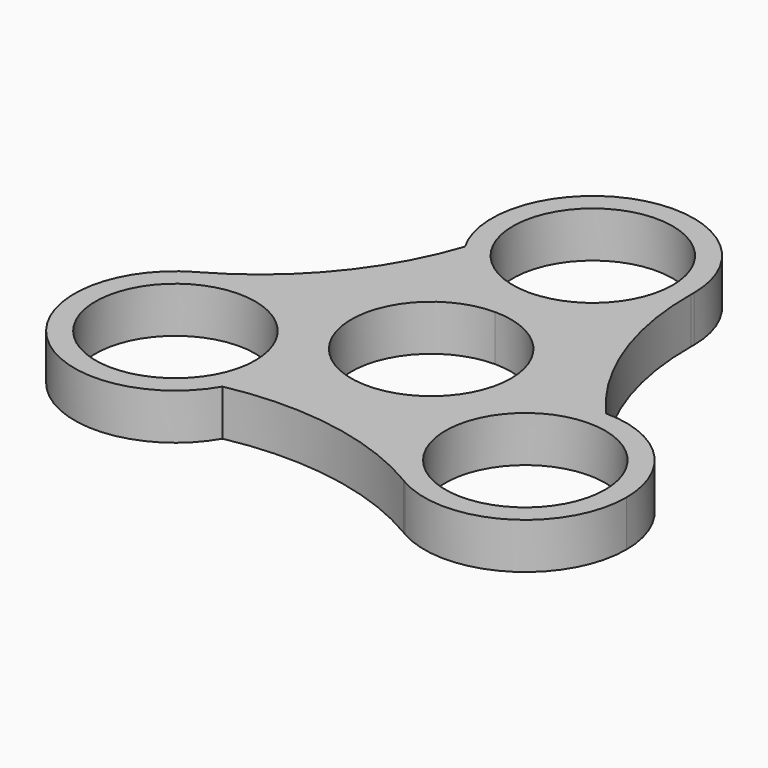
from build123d import *

# Parameters (mm, degrees)
F1_R     = 11.049
F2_DEPTH = 6.35


with BuildPart() as f2:
    # F1 (on face) → F2 (new body)
    with BuildSketch(Plane.XY):
        with BuildLine():
            ThreePointArc((13.9621660883, 27.472220007), (13.9654123098, 27.7061212363), (13.97, 27.94))
            ThreePointArc((13.97, 27.94), (-3.6157020601, 41.4339837933), (-12.0983748909, 20.955))
            ThreePointArc((-12.0983748909, 20.955), (-6.9849999951, 15.8416251063), (1.14e-08, 13.97))
            ThreePointArc((1.14e-08, 13.97), (9.7114883941, 17.8976948278), (13.9621660883, 27.472220007))
        make_face()
        with BuildLine():
            ThreePointArc((11.049, 27.94), (7.8128228253, 20.1271771747), (0, 16.891))
            ThreePointArc((0, 16.891), (-7.8128228253, 35.7528228253), (11.049, 27.94))
        make_face(mode=Mode.SUBTRACT)
        with BuildLine():
            ThreePointArc((1.14e-08, 13.97), (-6.9849999951, 15.8416251063), (-12.0983748909, 20.955))
            ThreePointArc((-12.0983748909, 20.955), (-19.3348001595, 7.9193573575), (-30.7727234686, -1.6445194791))
            ThreePointArc((-30.7727234686, -1.6445194791), (-20.3556031034, -0.5384516084), (-12.0983754336, -6.98499906))
            ThreePointArc((-12.0983754336, -6.98499906), (-12.0983746167, 6.9850004749), (1.14e-08, 13.97))
        make_face()
        with BuildLine():
            ThreePointArc((24.1967497817, 0), (16.525764733, 12.7847494365), (13.9621660883, 27.472220007))
            ThreePointArc((13.9621660883, 27.472220007), (9.7114883941, 17.8976948278), (1.14e-08, 13.97))
            ThreePointArc((1.14e-08, 13.97), (9.8782817372, 9.8782817292), (13.97, 0))
            ThreePointArc((13.97, 0), (13.4939839355, -3.6157015292), (12.0983754405, -6.984999048))
            ThreePointArc((12.0983754405, -6.984999048), (17.2117502577, -1.8716248343), (24.1967497817, 0))
        make_face()
        with BuildLine():
            ThreePointArc((13.97, 0), (9.8782817372, 9.8782817292), (1.14e-08, 13.97))
            ThreePointArc((1.14e-08, 13.97), (-12.0983746167, 6.9850004749), (-12.0983754336, -6.98499906))
            ThreePointArc((-12.0983754336, -6.98499906), (6.9e-09, -13.97), (12.0983754405, -6.984999048))
            ThreePointArc((12.0983754405, -6.984999048), (13.4939839355, -3.6157015292), (13.97, 0))
        make_face()
        with BuildLine():
            ThreePointArc((11.049, 0), (-7.8128228253, -7.8128228253), (0, 11.049))
            ThreePointArc((0, 11.049), (7.8128228253, 7.8128228253), (11.049, 0))
        make_face(mode=Mode.SUBTRACT)
        with BuildLine():
            ThreePointArc((-12.0983754336, -6.98499906), (-20.3556031034, -0.5384516084), (-30.7727234686, -1.6445194791))
            ThreePointArc((-30.7727234686, -1.6445194791), (-30.9769109858, -1.7586587835), (-31.1817497817, -1.8716251091))
            ThreePointArc((-31.1817497817, -1.8716251091), (-34.0750315149, -23.8482817332), (-12.0983748909, -20.955))
            ThreePointArc((-12.0983748909, -20.955), (-10.7027659885, -17.5857020601), (-10.2267497817, -13.97))
            ThreePointArc((-10.2267497817, -13.97), (-10.7027661289, -10.3542974157), (-12.0983754336, -6.98499906))
        make_face()
        with Locations((-24.1967497817, -13.97)):
            Circle(F1_R, mode=Mode.SUBTRACT)
        with BuildLine():
            ThreePointArc((38.1667497817, -13.97), (34.0750315149, -4.0917182668), (24.1967497817, 0))
            ThreePointArc((24.1967497817, 0), (17.2117502577, -1.8716248343), (12.0983754405, -6.984999048))
            ThreePointArc((12.0983754405, -6.984999048), (10.6441140583, -17.359242533), (16.8105573802, -25.8277005278))
            ThreePointArc((16.8105573802, -25.8277005278), (17.0114986761, -25.9474624527), (17.2117497817, -26.0683748909))
            ThreePointArc((17.2117497817, -26.0683748909), (31.1817497817, -26.0683748909), (38.1667497817, -13.97))
        make_face()
        with Locations((24.1967497817, -13.97)):
            Circle(F1_R, mode=Mode.SUBTRACT)
        with BuildLine():
            ThreePointArc((12.0983754405, -6.984999048), (6.9e-09, -13.97), (-12.0983754336, -6.98499906))
            ThreePointArc((-12.0983754336, -6.98499906), (-10.7027661289, -10.3542974157), (-10.2267497817, -13.97))
            ThreePointArc((-10.2267497817, -13.97), (-10.7027659885, -17.5857020601), (-12.0983748909, -20.955))
            ThreePointArc((-12.0983748909, -20.955), (2.8090354265, -20.704106794), (16.8105573802, -25.8277005278))
            ThreePointArc((16.8105573802, -25.8277005278), (10.6441140583, -17.359242533), (12.0983754405, -6.984999048))
        make_face()
    extrude(amount=F2_DEPTH)


solid = f2.part
